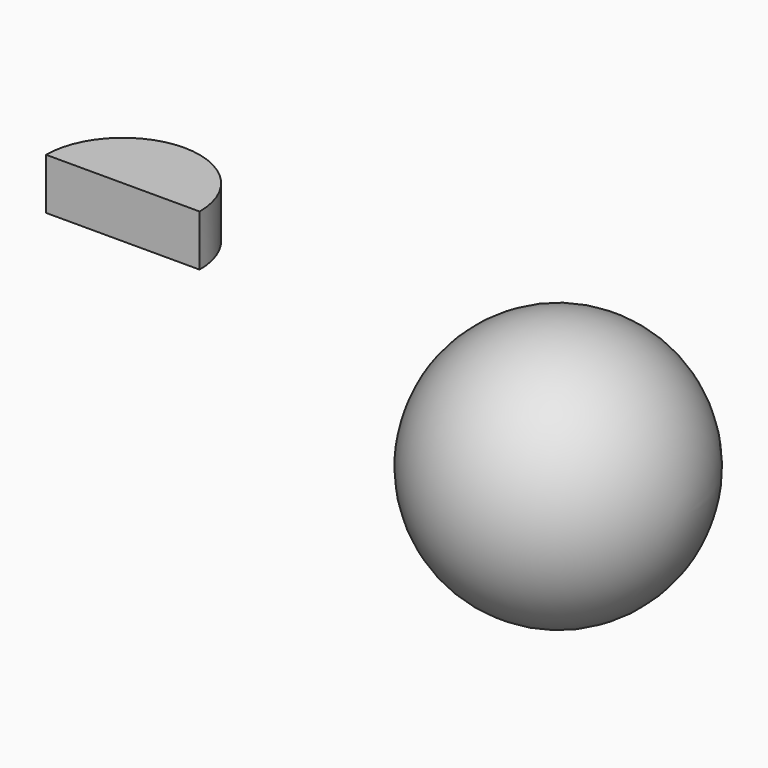
from build123d import *

# Parameters (mm, degrees)
F1_DEPTH = 25.4


with BuildPart() as f1:
    # F0 (on Top) → F1 (new body)
    with BuildSketch(Plane.XY):
        with BuildLine():
            Line((-44.8392927647, 35.3839807212), (-6.7392927647, 35.3839807212))
            ThreePointArc((-6.7392927647, 35.3839807212), (-17.8985244015, 62.3247490844), (-44.8392927647, 73.4839807212))
            Line((-44.8392927647, 73.4839807212), (-44.8392927647, 35.3839807212))
        make_face()
        with BuildLine():
            Line((-44.8392927647, 35.3839807212), (-44.8392927647, 73.4839807212))
            ThreePointArc((-44.8392927647, 73.4839807212), (-71.7800611279, 62.3247490844), (-82.9392927647, 35.3839807212))
            Line((-82.9392927647, 35.3839807212), (-44.8392927647, 35.3839807212))
        make_face()
    extrude(amount=F1_DEPTH)


with BuildPart() as f3:
    # F2 (on Top) → F3 (revolve)
    with BuildSketch(Plane.XY):
        with BuildLine():
            Line((141.4585729837, -6.7641003989), (268.4585729837, -6.7641003989))
            ThreePointArc((268.4585729837, -6.7641003989), (204.9585729837, 56.7358996011), (141.4585729837, -6.7641003989))
        make_face()
    revolve(axis=Axis((204.9585729837, -6.7641003989, 0), (1, 0, 0)))


solid = Compound([f1.part, f3.part])
